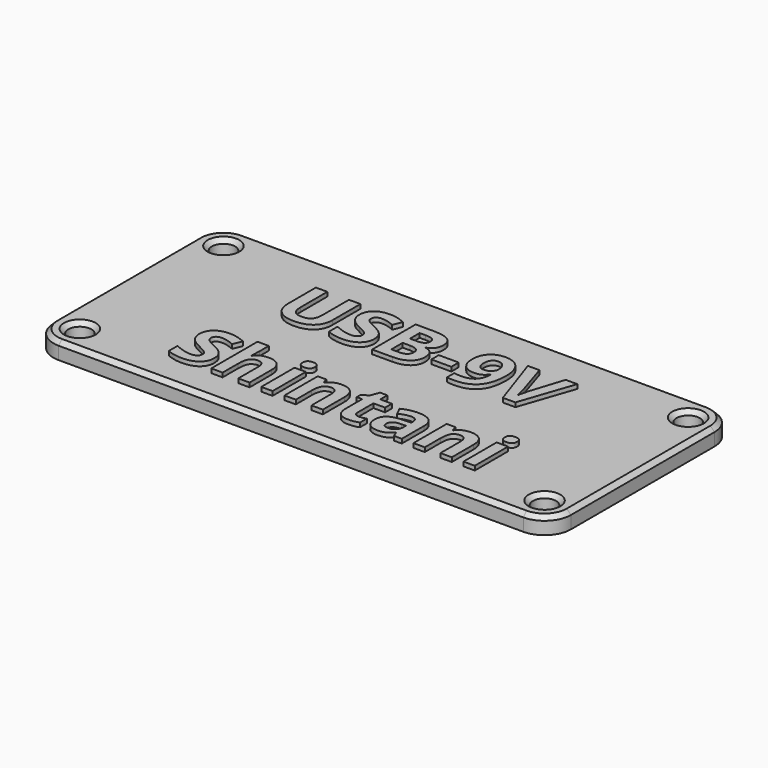
from build123d import *

# Parameters (mm, degrees)
F0_W         = 49
F0_H         = 22
F1_DEPTH     = 1.6
F2_R         = 2.5
F4_D         = 2.2
F5_SIZE      = 0.4
F6_TEXT_SIZE = 7.2039621792
F7_DEPTH     = 0.4


# Not quite as in the source:
# - Text() gives the source's letters only with a copy of the font that has no kerning and outlines rounded to 1/6400 em; it was checked with that copy


with BuildPart() as f1:
    # F0 (on Top) → F1 (new body)
    with BuildSketch(Plane.XY):
        with Locations((22.5, 9)):
            Rectangle(F0_W, F0_H)
    extrude(amount=F1_DEPTH)

    # F2
    f2_edges = [f1.edges().sort_by_distance(p)[0] for p in [
        (47, -2, 0.8),
        (47, 20, 0.8),
        (-2, 20, 0.8),
        (-2, -2, 0.8),
    ]]
    fillet(f2_edges, radius=F2_R)

    # F4 (through all)
    with Locations(Plane.XY.offset(1.6)):
        with Locations((44.5, 0.5), (44.5, 17.5), (0.5, 17.5), (0.5, 0.5)):
            Hole(F4_D / 2)

    # F5
    f5_edges = [f1.edges().sort_by_distance(p)[0] for p in [
        (47, 9, 1.6),
        (46.267767, -1.267767, 1.6),
        (46.267767, 19.267767, 1.6),
        (22.5, -2, 1.6),
        (22.5, 20, 1.6),
        (-1.267767, -1.267767, 1.6),
        (-1.267767, 19.267767, 1.6),
        (-2, 9, 1.6),
        (-0.6, 0.5, 1.6),
        (43.4, 0.5, 1.6),
        (-0.6, 17.5, 1.6),
        (43.4, 17.5, 1.6),
    ]]
    chamfer(f5_edges, length=F5_SIZE)

    # F6 (on face) → F7 (join)
    with BuildSketch(Plane.XY.offset(1.6)):
        with Locations((9.8719045475, 10.813147231)):
            Text('USB-9V', F6_TEXT_SIZE, font='Open Sans', font_style=FontStyle.BOLD, text_align=(TextAlign.LEFT, TextAlign.BOTTOM))
        with Locations((8, 1.0157586673)):
            Text('Shintani', F6_TEXT_SIZE, font='Open Sans', font_style=FontStyle.BOLD, text_align=(TextAlign.LEFT, TextAlign.BOTTOM))
    extrude(amount=F7_DEPTH)


solid = f1.part
